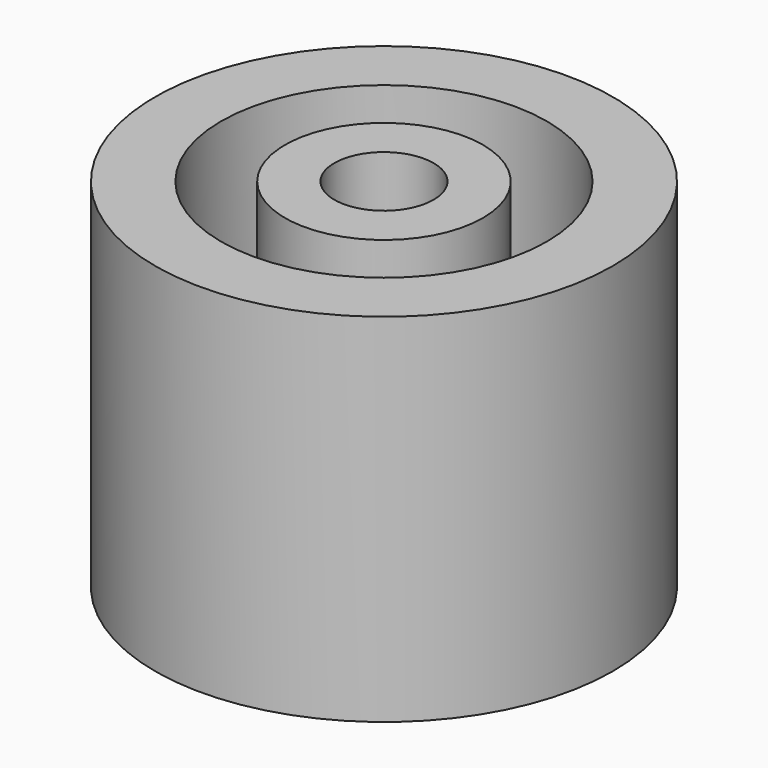
from build123d import *

# Parameters (mm, degrees)
F0_R     = 9.623
F1_DEPTH = 15
F2_R     = 2.0875
F3_DEPTH = 10
F2_R_2   = 6.85
F2_R_3   = 4.1625
F4_DEPTH = 10


# Not quite as in the source:
# - a feature names something its author has since deleted; it is built from what else it names


with BuildPart() as f1:
    # F0 (on Top) → F1 (new body)
    with BuildSketch(Plane.XY):
        Circle(F0_R)
    extrude(amount=F1_DEPTH)

    # F2 (on face) → F3 (cut)
    with BuildSketch(Plane.XY.offset(15)):
        Circle(F2_R)
    extrude(amount=-F3_DEPTH, mode=Mode.SUBTRACT)

    # F2 (on face) → F4 (cut)
    with BuildSketch(Plane.XY.offset(15)):
        Circle(F2_R_2)
        Circle(F2_R_3, mode=Mode.SUBTRACT)
    extrude(amount=-F4_DEPTH, mode=Mode.SUBTRACT)


solid = f1.part
